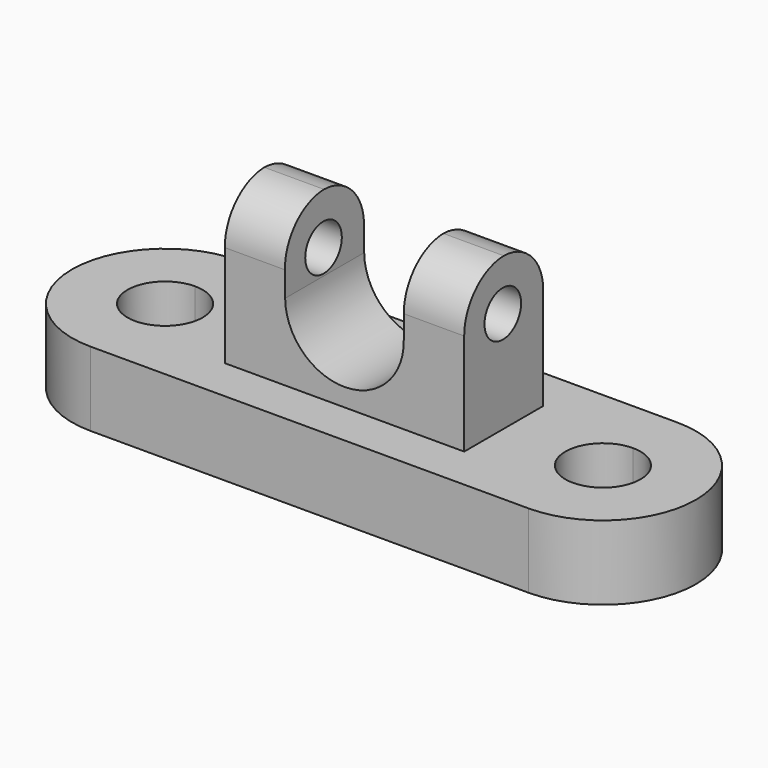
from build123d import *

# Parameters (mm, degrees)
F1_DEPTH    = 9.906
F2_W        = 31.9448374212
F2_H        = 13.18457257
F3_DEPTH    = 20.32
F5_DEPTH    = 25.4
F6_T1_DEPTH = 41.6882551367
F6_T3_DEPTH = 41.7866267939
F7_R        = 3.0503938931
F8_DEPTH    = 57.5943291351


# Not quite as in the source:
# - a fillet or chamfer that OpenCascade refuses, or shapes differently, is made with other operations: its cross-section is extruded or revolved along the edge and cut away or added


with BuildPart() as f1:
    # F0 (on Top) → F1 (new body)
    with BuildSketch(Plane.XY):
        with BuildLine():
            Line((-29.21, -12.4109104246), (29.21, -12.4109104246))
            Line((29.21, -12.4109104246), (29.21, -5.0137877216))
            ThreePointArc((29.21, -5.0137877216), (24.1962122784, 0), (29.21, 5.0137877216))
            Line((29.21, 5.0137877216), (29.21, 12.4109104246))
            Line((29.21, 12.4109104246), (-29.21, 12.4109104246))
            Line((-29.21, 12.4109104246), (-29.21, 5.0137877216))
            ThreePointArc((-29.21, 5.0137877216), (-25.6647167027, 3.5452832973), (-24.1962122784, 0))
            ThreePointArc((-24.1962122784, 0), (-25.6647167027, -3.5452832973), (-29.21, -5.0137877216))
            Line((-29.21, -5.0137877216), (-29.21, -12.4109104246))
        make_face()
        with BuildLine():
            ThreePointArc((-29.21, 12.4109104246), (-41.6209104246, 0), (-29.21, -12.4109104246))
            Line((-29.21, -12.4109104246), (-29.21, -5.0137877216))
            ThreePointArc((-29.21, -5.0137877216), (-34.2237877216, 0), (-29.21, 5.0137877216))
            Line((-29.21, 5.0137877216), (-29.21, 12.4109104246))
        make_face()
        with BuildLine():
            Line((29.21, -5.0137877216), (29.21, -12.4109104246))
            ThreePointArc((29.21, -12.4109104246), (41.6209104246, 0), (29.21, 12.4109104246))
            Line((29.21, 12.4109104246), (29.21, 5.0137877216))
            ThreePointArc((29.21, 5.0137877216), (32.7552832973, 3.5452832973), (34.2237877216, 0))
            ThreePointArc((34.2237877216, 0), (32.7552832973, -3.5452832973), (29.21, -5.0137877216))
        make_face()
    extrude(amount=F1_DEPTH)

    # F2 (on face) → F3 (join)
    with BuildSketch(Plane.XY.offset(9.906)):
        Rectangle(F2_W, F2_H)
    extrude(amount=F3_DEPTH)

    # F4 (on face) → F5 (cut)
    with BuildSketch(Plane.XZ.offset(6.592286285)):
        with BuildLine():
            Line((-8.0107270402, 30.226), (-7.9157502647, 20.1440832174))
            ThreePointArc((-7.9157502647, 20.1440832174), (0.1590473721, 12.3041500236), (7.912355383, 20.462159845))
            Line((7.912355383, 20.462159845), (7.912355383, 30.226))
            Line((7.912355383, 30.226), (-8.0107270402, 30.226))
        make_face()
    extrude(amount=-F5_DEPTH, mode=Mode.SUBTRACT)

    # F6: fillet of radius 6.7453126933 on 4 edges, made by hand

    # F6_s2 → F6_t1 (cut)
    with BuildSketch(Plane.YZ.offset(-32.8357004438)):
        with BuildLine():
            ThreePointArc((-6.592286285, 23.4806873067), (-4.6166299384, 28.2503436534), (0.1530264083, 30.226))
            Line((0.1530264083, 30.226), (-6.592286285, 30.226))
            Line((-6.592286285, 30.226), (-6.592286285, 23.4806873067))
        make_face()
        with BuildLine():
            ThreePointArc((6.592286285, 23.4806873067), (4.6166299384, 28.2503436534), (-0.1530264083, 30.226))
            Line((-0.1530264083, 30.226), (6.592286285, 30.226))
            Line((6.592286285, 30.226), (6.592286285, 23.4806873067))
        make_face()
    extrude(amount=F6_T1_DEPTH, mode=Mode.SUBTRACT)

    # F6_s4 → F6_t3 (cut)
    with BuildSketch(Plane.YZ.offset(-8.9509263502)):
        with BuildLine():
            ThreePointArc((-6.592286285, 23.4806873067), (-4.6166299384, 28.2503436534), (0.1530264083, 30.226))
            Line((0.1530264083, 30.226), (-6.592286285, 30.226))
            Line((-6.592286285, 30.226), (-6.592286285, 23.4806873067))
        make_face()
        with BuildLine():
            ThreePointArc((6.592286285, 23.4806873067), (4.6166299384, 28.2503436534), (-0.1530264083, 30.226))
            Line((-0.1530264083, 30.226), (6.592286285, 30.226))
            Line((6.592286285, 30.226), (6.592286285, 23.4806873067))
        make_face()
    extrude(amount=F6_T3_DEPTH, mode=Mode.SUBTRACT)

    # F7 (on face) → F8 (cut, through all)
    with BuildSketch(Plane(origin=(-15.9724187106, 0, 0), x_dir=(0, -1, 0), z_dir=(-1, 0, 0))):
        with Locations((0.1530264083, 23.4806873067)):
            Circle(F7_R)
    extrude(amount=-F8_DEPTH, mode=Mode.SUBTRACT)


solid = f1.part
